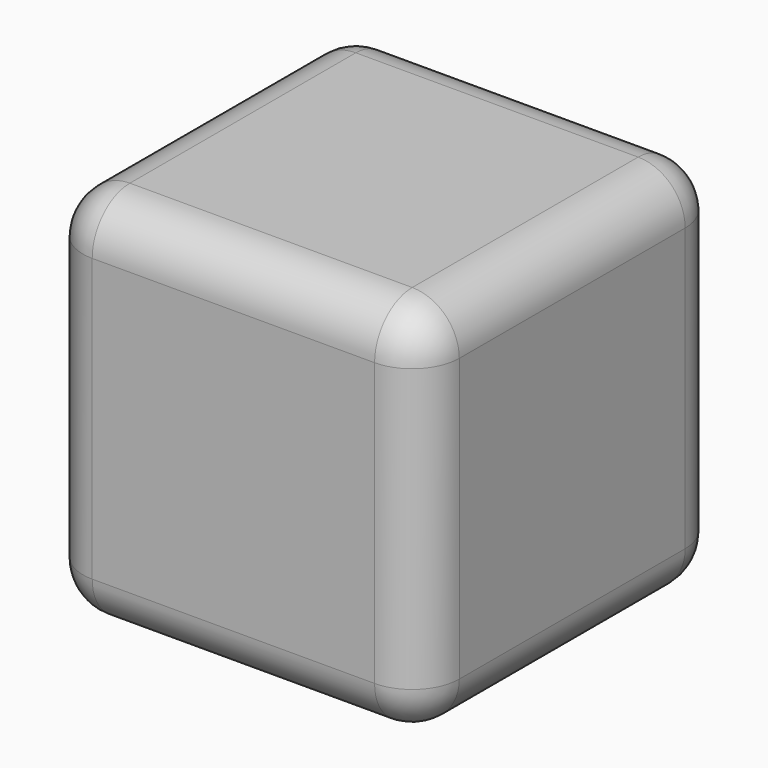
from build123d import *

# Parameters (mm, degrees)
F0_W         = 16
F0_H         = 16
F1_DEPTH     = 16
F2_R         = 2
F3_T1_DEPTH  = 12
F3_S5_W      = 2
F3_S5_H      = 2
F3_T6_DEPTH  = 2
F3_S11_W     = 2
F3_S11_H     = 2
F3_T12_DEPTH = 2


# Not quite as in the source:
# - a fillet or chamfer that OpenCascade refuses, or shapes differently, is made with other operations: its cross-section is extruded or revolved along the edge and cut away or added


with BuildPart() as f1:
    # F0 (on Front) → F1 (new body)
    with BuildSketch(Plane.XZ):
        Rectangle(F0_W, F0_H)
    extrude(amount=F1_DEPTH)

    # F2
    f2_edges = [f1.edges().sort_by_distance(p)[0] for p in [
        (0, -16, 8),
        (8, -8, 8),
        (8, -8, -8),
        (-8, -16, 0),
        (8, 0, 0),
        (8, -16, 0),
        (-8, -8, -8),
        (-8, -8, 8),
        (-8, 0, 0),
        (0, 0, 8),
        (0, 0, -8),
    ]]
    fillet(f2_edges, radius=F2_R)

    # F3: fillet of radius 2 on 1 edges, made by hand

    # F3_s2 → F3_t1 (cut)
    with BuildSketch(Plane.YZ.offset(-6)):
        with BuildLine():
            ThreePointArc((-16, -6), (-15.4142135624, -7.4142135624), (-14, -8))
            Line((-14, -8), (-16, -8))
            Line((-16, -8), (-16, -6))
        make_face()
    extrude(amount=F3_T1_DEPTH, mode=Mode.SUBTRACT)


with BuildPart() as f3_tool4:
    # F3_s5 → F3_t6 (new body)
    with BuildSketch(Plane.XZ.offset(14)):
        with Locations((-7, -7)):
            Rectangle(F3_S5_W, F3_S5_H)
    extrude(amount=F3_T6_DEPTH)

    # F3_s7 → F3_t8 (revolve, cut)
    with BuildSketch(Plane(origin=(-6, -14, -6), x_dir=(0.7071067812, 0, 0.7071067812), z_dir=(0.7071067812, 0, -0.7071067812))):
        with BuildLine():
            ThreePointArc((0, -2), (2, 0), (0, 2))
            Line((0, 2), (0, -2))
        make_face()
    revolve(axis=Axis((-6, -14, -6), (0, -1, 0)), mode=Mode.SUBTRACT)


with BuildPart() as f1_1:
    add(f1.part)

    # F3_t3: cut F3_tool4
    add(f3_tool4.part, mode=Mode.SUBTRACT)


with BuildPart() as f3_tool10:
    # F3_s11 → F3_t12 (new body)
    with BuildSketch(Plane.XZ.offset(14)):
        with Locations((7, -7)):
            Rectangle(F3_S11_W, F3_S11_H)
    extrude(amount=F3_T12_DEPTH)

    # F3_s13 → F3_t14 (revolve, cut)
    with BuildSketch(Plane(origin=(6, -14, -6), x_dir=(-0.7071067812, 0, 0.7071067812), z_dir=(0.7071067812, 0, 0.7071067812))):
        with BuildLine():
            ThreePointArc((0, -2), (2, 0), (0, 2))
            Line((0, 2), (0, -2))
        make_face()
    revolve(axis=Axis((6, -14, -6), (0, -1, 0)), mode=Mode.SUBTRACT)


with BuildPart() as f1_2:
    add(f1_1.part)

    # F3_t9: cut F3_tool10
    add(f3_tool10.part, mode=Mode.SUBTRACT)


solid = f1_2.part
